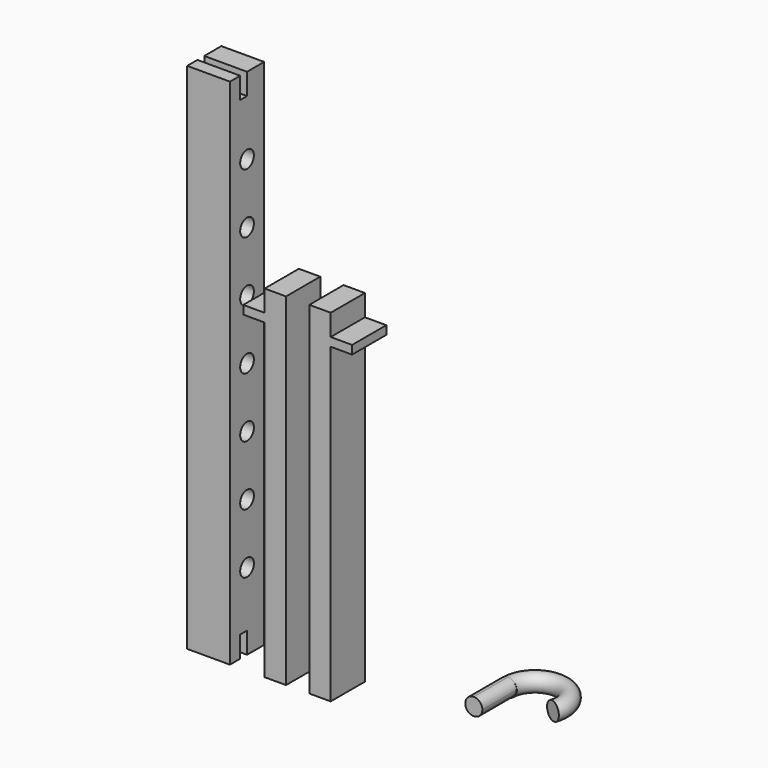
from build123d import *

# Parameters (mm, degrees)
F0_W      = 6.35
F0_H      = 12.7
F1_DEPTH  = 101.6
F2_W      = 12.7
F2_H      = 2.54
F3_DEPTH  = 6.35
F4_W      = 12.7
F4_H      = 2.54
F5_DEPTH  = 6.35
F6_W      = 12.7
F6_H      = 12.7
F7_DEPTH  = 152.4
F8_W      = 12.7
F8_H      = 2.54
F9_DEPTH  = 6.35
F10_W     = 12.7
F10_H     = 2.54
F11_DEPTH = 6.35
F12_R     = 2.54
F13_DEPTH = 12.7
F14_W     = 5.08
F14_H     = 12.7
F15_DEPTH = 5.08
F16_R     = 2.53999
F18_R     = 2.6317001642
F19_ANGLE = 200


# Not quite as in the source:
# - a fillet or chamfer is up to 0.001 mm smaller than in the source, because OpenCascade refuses the exact size


with BuildPart() as f1:
    # F0 (on Top) → F1 (new body)
    with BuildSketch(Plane.XY):
        with Locations((-7.2030832142, -35.1877281606)):
            Rectangle(F0_W, F0_H)
    extrude(amount=F1_DEPTH)

    # F4 (on face) → F5 (join)
    with BuildSketch(Plane(origin=(-10.3780832142, 0, 0), x_dir=(0, -1, 0), z_dir=(-1, 0, 0))):
        with Locations((35.1877281606, 93.98)):
            Rectangle(F4_W, F4_H)
    extrude(amount=F5_DEPTH)


with BuildPart() as f1b:
    # F0 (on Top) → F1, piece 2 (new body)
    with BuildSketch(Plane.XY):
        with Locations((6.0000692412, -35.1179832757)):
            Rectangle(F0_W, F0_H)
    extrude(amount=F1_DEPTH)

    # F2 (on face) → F3 (join)
    with BuildSketch(Plane.YZ.offset(9.1750692412)):
        with Locations((-35.1179832757, 93.98)):
            Rectangle(F2_W, F2_H)
    extrude(amount=F3_DEPTH)


with BuildPart() as f7:
    # F6 (on Top) → F7 (new body)
    with BuildSketch(Plane.XY):
        with Locations((-26.9454600453, -35.3058190852)):
            Rectangle(F6_W, F6_H)
    extrude(amount=F7_DEPTH)

    # F8 (on face) → F9 (cut)
    with BuildSketch(Plane.XY.offset(152.4)):
        with Locations((-26.9454600453, -36.5758190852)):
            Rectangle(F8_W, F8_H)
    extrude(amount=-F9_DEPTH, mode=Mode.SUBTRACT)

    # F10 (on face) → F11 (cut)
    with BuildSketch(Plane(origin=(0, 0, 0), x_dir=(1, 0, 0), z_dir=(0, 0, -1))):
        with Locations((-26.9454600453, 36.5758190852)):
            Rectangle(F10_W, F10_H)
    extrude(amount=-F11_DEPTH, mode=Mode.SUBTRACT)

    # F12 (on face) → F13 (cut)
    with BuildSketch(Plane(origin=(-33.2954600453, 0, 0), x_dir=(0, -1, 0), z_dir=(-1, 0, 0))):
        with Locations((35.3058190852, 22.86)):
            Circle(F12_R)
        with Locations((35.3058190852, 40.64)):
            Circle(F12_R)
        with Locations((35.3058190852, 76.2)):
            Circle(F12_R)
        with Locations((35.3058190852, 93.98)):
            Circle(F12_R)
        with Locations((35.3058190852, 111.76)):
            Circle(F12_R)
        with Locations((35.3058190852, 58.42)):
            Circle(F12_R)
        with Locations((35.3058190852, 129.54)):
            Circle(F12_R)
    extrude(amount=-F13_DEPTH, mode=Mode.SUBTRACT)


with BuildPart() as f15:
    # F14 (on Top) → F15 (new body)
    with BuildSketch(Plane.XY):
        with Locations((39.7342580192, -20.1999229612)):
            Rectangle(F14_W, F14_H)
    extrude(amount=F15_DEPTH)

    # F16 (radius 2.54 in the source; OpenCascade refuses exactly that, so slightly less here)
    f16_edges = [f15.edges().sort_by_distance(p)[0] for p in [
        (42.274258, -20.199923, 5.08),
        (37.194258, -20.199923, 5.08),
        (42.274258, -20.199923, 0),
        (37.194258, -20.199923, 0),
    ]]
    fillet(f16_edges, radius=F16_R)

    # F18 (on offset) → F19 (revolve)
    with BuildSketch(Plane(origin=(0, -13.8499229612, 0), x_dir=(-1, 0, 0), z_dir=(0, 1, 0))):
        with Locations((-39.7273041308, 2.3956361692)):
            Circle(F18_R)
    revolve(axis=Axis((47.7343313396, -13.8499229612, 0.46519842), (0, 0, -1)), revolution_arc=F19_ANGLE)


solid = Compound([f1.part, f1b.part, f7.part, f15.part])
